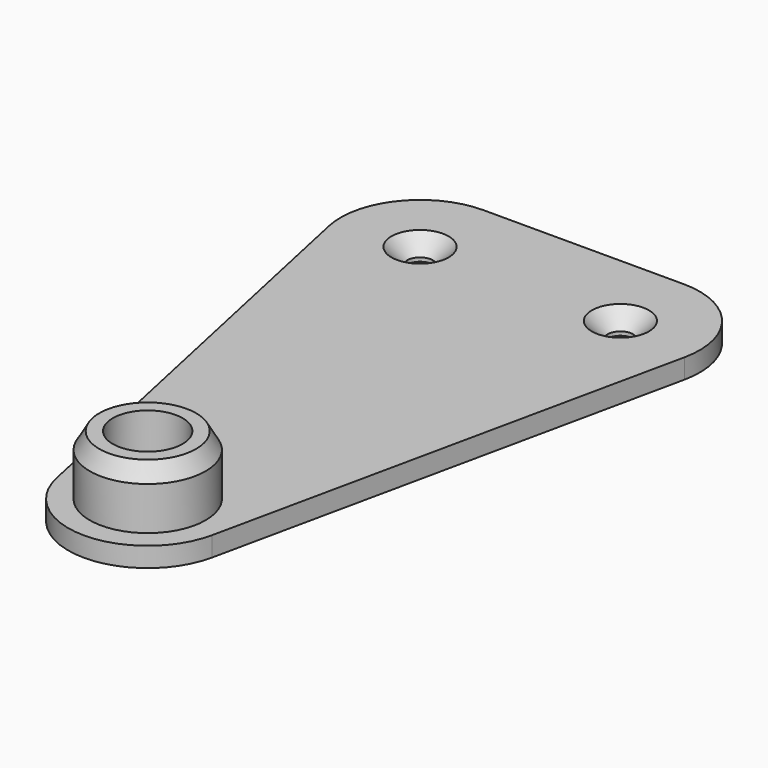
from build123d import *

# Parameters (mm, degrees)
F0_R     = 4.6355
F0_R_2   = 1.016
F1_DEPTH = 1.5748
F0_R_3   = 2.794
F2_DEPTH = 6.35
F3_SIZE  = 1.27


# Not quite as in the source:
# - a fillet or chamfer that OpenCascade refuses, or shapes differently, is made with other operations: its cross-section is extruded or revolved along the edge and cut away or added
# - a feature names something its author has since deleted; it is built from what else it names


with BuildPart() as f1:
    # F0 (on Top) → F1 (new body)
    with BuildSketch(Plane.XY):
        with BuildLine():
            Line((-14.2215059748, 35.912132599), (-6.2079540965, -1.3355919797))
            ThreePointArc((-6.2079540965, -1.3355919797), (0, -6.35), (6.2079540965, -1.3355919797))
            Line((6.2079540965, -1.3355919797), (14.2215059748, 35.912132599))
            ThreePointArc((14.2215059748, 35.912132599), (12.9533650869, 41.2378054632), (8.0135518783, 43.5977245787))
            Line((8.0135518783, 43.5977245787), (-8.0135518783, 43.5977245787))
            ThreePointArc((-8.0135518783, 43.5977245787), (-12.9533650869, 41.2378054632), (-14.2215059748, 35.912132599))
        make_face()
        Circle(F0_R, mode=Mode.SUBTRACT)
        with Locations((-8.0135518783, 37.2477245787)):
            Circle(F0_R_2, mode=Mode.SUBTRACT)
        with Locations((8.0135518783, 37.2477245787)):
            Circle(F0_R_2, mode=Mode.SUBTRACT)
    extrude(amount=F1_DEPTH)

    # F0 (on Top) → F2 (join)
    with BuildSketch(Plane.XY):
        Circle(F0_R)
        Circle(F0_R_3, mode=Mode.SUBTRACT)
    extrude(amount=F2_DEPTH)

    # F3
    f3_edges = [f1.edges().sort_by_distance(p)[0] for p in [
        (-9.029552, 37.247725, 1.5748),
        (6.997552, 37.247725, 1.5748),
    ]]
    chamfer(f3_edges, length=F3_SIZE)

    # F4: chamfer of 0.762 x 1.3198227154 on 1 edges, made by hand

    # F4_s1 → F4_t2 (revolve, cut)
    with BuildSketch(Plane.XZ):
        Polygon((4.6355, 5.0301772846), (3.8735, 6.35), (4.6355, 6.35), align=None)
    revolve(axis=Axis((0, 0, 6.35), (0, 0, 1)), mode=Mode.SUBTRACT)


solid = f1.part
